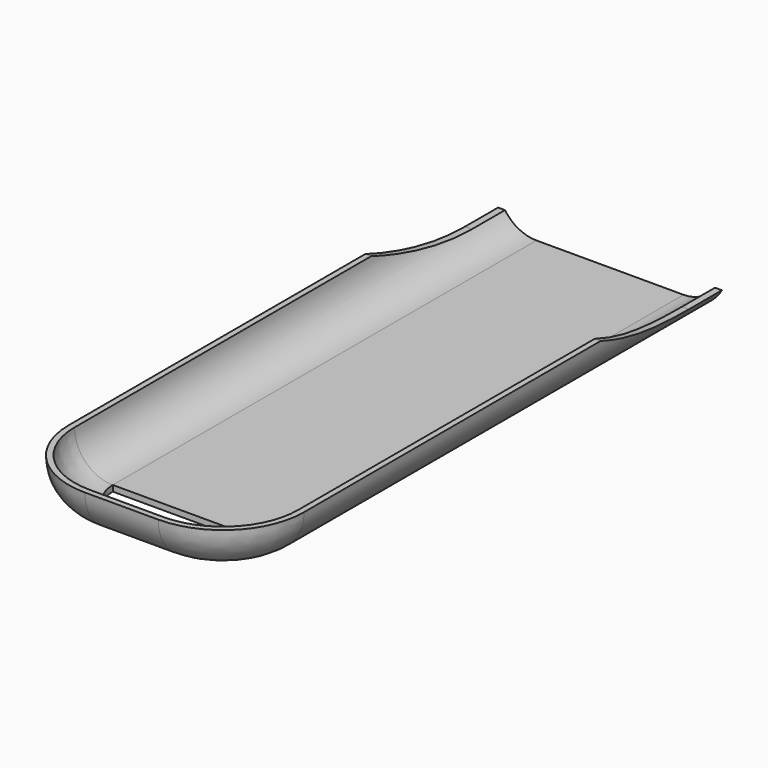
from build123d import *

# Parameters (mm, degrees)
F0_W     = 80
F0_H     = 180
F1_DEPTH = 15
F2_W     = 50
F2_H     = 2
F3_DEPTH = 180
F4_ANGLE = 90
F5_ANGLE = 90
F6_DEPTH = 25
F9_DEPTH = 80.001


with BuildPart() as f1:
    # F0 (on Top) → F1 (new body)
    with BuildSketch(Plane.XY):
        Rectangle(F0_W, F0_H)
    extrude(amount=F1_DEPTH)

    # F2 (on face) → F3 (intersect, through all)
    with BuildSketch(Plane.XZ.offset(90)):
        with BuildLine():
            Line((-38, 15), (-40, 15))
            ThreePointArc((-40, 15), (-35.6066017178, 4.3933982822), (-25, 0))
            Line((-25, 0), (-25, 2))
            ThreePointArc((-25, 2), (-34.1923881554, 5.8076118446), (-38, 15))
        make_face()
        with Locations((0, 1)):
            Rectangle(F2_W, F2_H)
        with BuildLine():
            Line((25, 2), (25, 0))
            ThreePointArc((25, 0), (35.6066017178, 4.3933982822), (40, 15))
            Line((40, 15), (38, 15))
            ThreePointArc((38, 15), (34.1923881554, 5.8076118446), (25, 2))
        make_face()
    extrude(amount=-F3_DEPTH, mode=Mode.INTERSECT)

    # F2 (on face) → F4 (revolve)
    with BuildSketch(Plane.XZ.offset(90)):
        with BuildLine():
            Line((25, 2), (25, 0))
            ThreePointArc((25, 0), (35.6066017178, 4.3933982822), (40, 15))
            Line((40, 15), (38, 15))
            ThreePointArc((38, 15), (34.1923881554, 5.8076118446), (25, 2))
        make_face()
    revolve(axis=Axis((12.5, -90, 8.5), (0, 0, -1)), revolution_arc=F4_ANGLE)

    # F2 (on face) → F5 (revolve)
    with BuildSketch(Plane.XZ.offset(90)):
        with BuildLine():
            Line((-38, 15), (-40, 15))
            ThreePointArc((-40, 15), (-35.6066017178, 4.3933982822), (-25, 0))
            Line((-25, 0), (-25, 2))
            ThreePointArc((-25, 2), (-34.1923881554, 5.8076118446), (-38, 15))
        make_face()
    revolve(axis=Axis((-12.5, -90, 8.5), (0, 0, 1)), revolution_arc=F5_ANGLE)

    # F6 (add, through all): a face of the model
    f6_faces = [f1.faces().sort_by_distance(p)[0] for p in [
        (-12.5, -111.8423881554, 5.6576118446),
    ]]
    extrude(f6_faces, amount=F6_DEPTH)

    # F8 (on face) → F9 (cut, through all)
    with BuildSketch(Plane.YZ.offset(40)):
        with BuildLine():
            Line((90, 7.6), (90, 15))
            Line((90, 15), (36, 15))
            ThreePointArc((36, 15), (55.6606293116, 9.4655638465), (76, 7.6))
            Line((76, 7.6), (90, 7.6))
        make_face()
    extrude(amount=-F9_DEPTH, mode=Mode.SUBTRACT)


solid = f1.part
